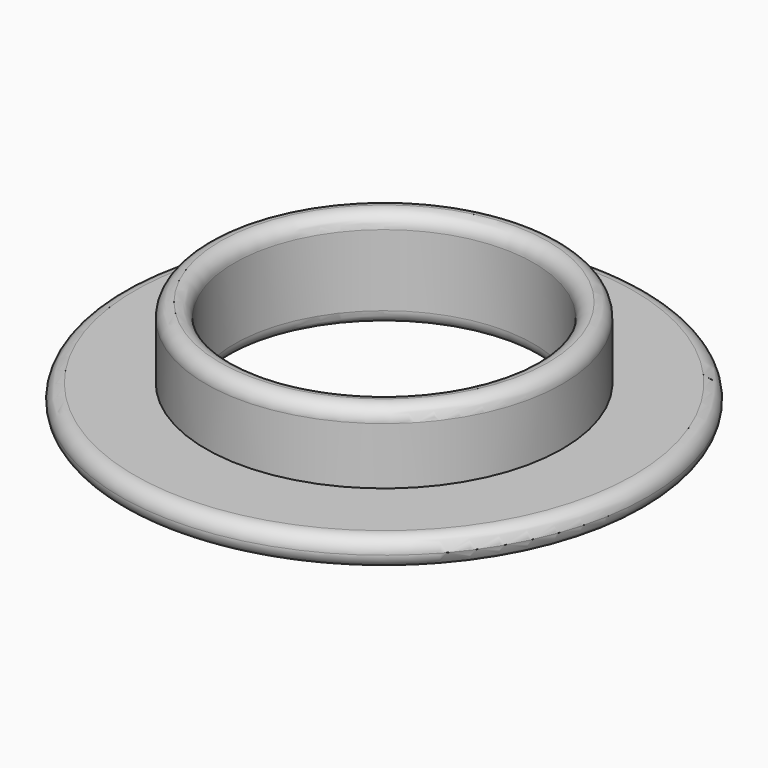
from build123d import *

# Parameters (mm, degrees)
F0_R     = 18.5
F1_DEPTH = 2
F2_R     = 12.5
F3_DEPTH = 5
F4_R     = 10.5
F5_DEPTH = 25
F6_R     = 1
F7_R     = 0.99999
F8_R     = 0.99999


# Not quite as in the source:
# - a fillet or chamfer is up to 0.001 mm smaller than in the source, because OpenCascade refuses the exact size


with BuildPart() as f1:
    # F0 (on Top) → F1 (new body)
    with BuildSketch(Plane.XY):
        Circle(F0_R)
    extrude(amount=F1_DEPTH)

    # F2 (on face) → F3 (join)
    with BuildSketch(Plane.XY.offset(2)):
        Circle(F2_R)
    extrude(amount=F3_DEPTH)

    # F4 (on face) → F5 (cut)
    with BuildSketch(Plane.XY.offset(7)):
        Circle(F4_R)
    extrude(amount=-F5_DEPTH, mode=Mode.SUBTRACT)

    # F6
    f6_edges = [f1.edges().sort_by_distance(p)[0] for p in [
        (-18.5, 0, 0),
        (-10.5, 0, 0),
    ]]
    fillet(f6_edges, radius=F6_R)

    # F7 (radius 1 in the source; OpenCascade refuses exactly that, so slightly less here)
    f7_edges = [f1.edges().sort_by_distance(p)[0] for p in [
        (-12.5, 0, 7),
        (-10.5, 0, 7),
    ]]
    fillet(f7_edges, radius=F7_R)

    # F8 (radius 1 in the source; OpenCascade refuses exactly that, so slightly less here)
    f8_edges = [f1.edges().sort_by_distance(p)[0] for p in [
        (-18.5, 0, 2),
    ]]
    fillet(f8_edges, radius=F8_R)


solid = f1.part
